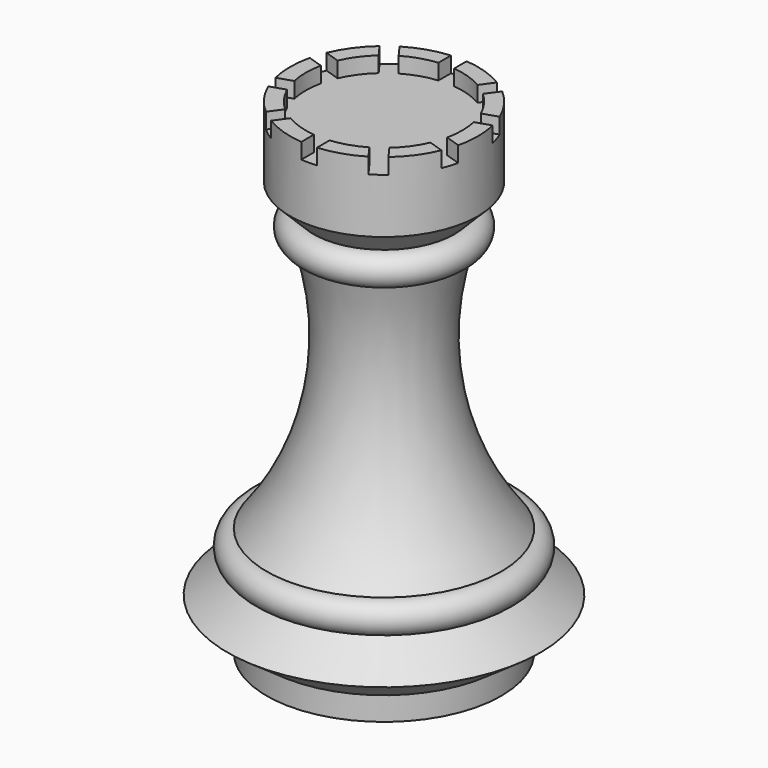
from build123d import *

# Parameters (mm, degrees)
F2_W            = 2.54
F2_H            = 2.54
F3_DEPTH        = 25.401
F3_DEPTH_BACK   = 25.4
F3_COPIES_COUNT = 5
F3_COPIES_ANGLE = 144


# Not quite as in the source:
# - a pattern or mirror of a feature is missing from the dataset's text; its kind, count and spacing are read off the source's solid


with BuildPart() as f1:
    # F0 (on Front) → F1 (revolve)
    with BuildSketch(Plane.XZ):
        with BuildLine():
            Line((0, 76.2), (0, 0))
            Line((0, 0), (19.05, 0))
            Line((19.05, 0), (19.05, 3.81))
            Line((19.05, 3.81), (25.4, 8.255))
            Line((25.4, 8.255), (19.05, 12.7))
            ThreePointArc((19.05, 12.7), (21.59, 15.24), (19.05, 17.78))
            ThreePointArc((19.05, 17.78), (10.2268710231, 37.1600383168), (11.43, 58.42))
            ThreePointArc((11.43, 58.42), (13.97, 60.96), (11.43, 63.5))
            Line((11.43, 63.5), (15.24, 67.31))
            Line((15.24, 67.31), (15.24, 78.74))
            Line((15.24, 78.74), (12.7, 78.74))
            Line((12.7, 78.74), (12.7, 76.2))
            Line((12.7, 76.2), (0, 76.2))
        make_face()
    revolve(axis=Axis((0, 0, 38.1), (0, 0, 1)))

    # F2 (on Front) → F3 (cut, two sides)
    with BuildSketch(Plane.XZ) as f3_sk:
        with Locations((0, 77.47)):
            Rectangle(F2_W, F2_H)
    f3 = extrude(amount=-F3_DEPTH, mode=Mode.SUBTRACT) + extrude(f3_sk.sketch, amount=F3_DEPTH_BACK, mode=Mode.SUBTRACT)

    # F3_copies: F3 ×5 about axis
    f3_copies_axis = Axis((0, 0, 0), (0, 0, 1))
    for i in range(1, F3_COPIES_COUNT):
        add(f3.rotate(f3_copies_axis, i * F3_COPIES_ANGLE / (F3_COPIES_COUNT - 1)), mode=Mode.SUBTRACT)


solid = f1.part
